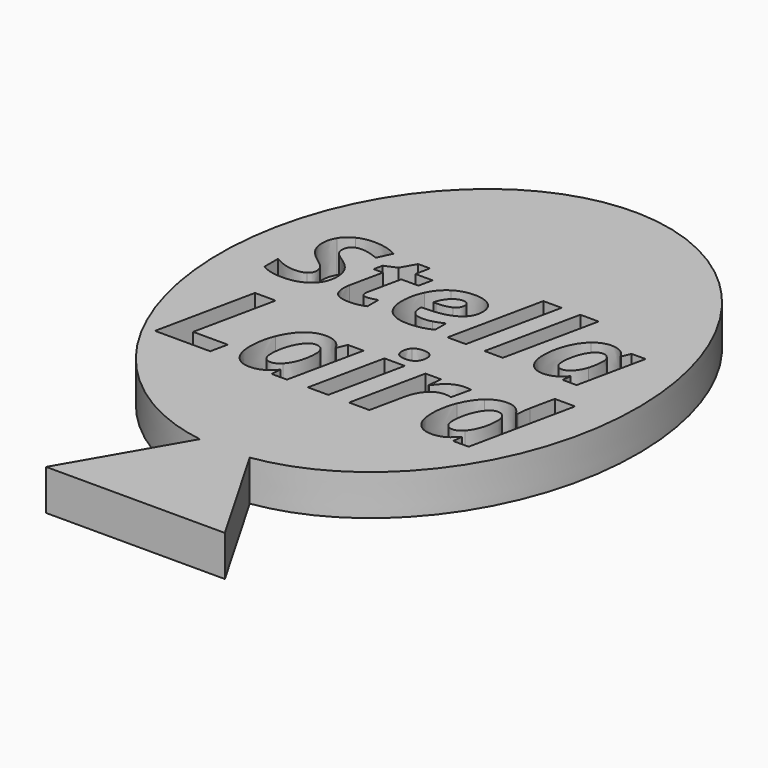
from build123d import *

# Parameters (mm, degrees)
F1_DEPTH       = 6.35
F0_TEXT_SIZE   = 19.5004373789
F0_TEXT_SIZE_2 = 21.6683653704
F2_DEPTH       = 1.27


# Not quite as in the source:
# - Text() gives the source's letters only with a copy of the font that has no kerning and outlines rounded to 1/6400 em; it was checked with that copy


with BuildPart() as f1:
    # F0 (on Top) → F1 (new body)
    with BuildSketch(Plane.XY):
        with BuildLine():
            add(Edge.make_bspline(
                [(3.9012639568, -39.93374284), (34.4777247718, -35.4132794138), (32.6371018831, 2.4039067683), (30.7964789943, 40.2210929505), (0, 40.2210929505)],
                knots=[3.2611985656, 3.2611985656, 3.2611985656, 4.7721919364, 4.7721919364, 6.2831853072, 6.2831853072, 6.2831853072], degree=2, weights=[1, 0.7279310805, 1, 0.7279310805, 1]))
            add(Edge.make_bspline(
                [(0, 40.2210929505), (-30.7964789943, 40.2210929505), (-32.6371018831, 2.4039067683), (-34.4777247718, -35.4132794138), (-3.9012639568, -39.93374284)],
                knots=[0, 0, 0, 1.5109933708, 1.5109933708, 3.0219867416, 3.0219867416, 3.0219867416], degree=2, weights=[1, 0.7279310805, 1, 0.7279310805, 1]))
            Line((-3.9012639568, -39.93374284), (0, -33.1765554531))
            Line((0, -33.1765554531), (3.9012639568, -39.93374284))
        make_face()
        Polygon((-17.4413733836, -20.9845771347), (-26.0850197571, -20.9845771347), (-22.8178365411, -5.5153956695), (-19.5777387818, -5.5153956695), (-22.2862844531, -18.2760314634), (-16.8691931105, -18.2760314634), align=None, mode=Mode.SUBTRACT)
        with BuildLine():
            add(Edge.make_bspline(
                [(-7.7481655624, -19.4508631483), (-9.1667663577, -21.1978751063), (-11.1236906053, -21.1978751063)],
                knots=[0, 0, 0, 1, 1, 1], degree=2))
            add(Edge.make_bspline(
                [(-11.1236906053, -21.1978751063), (-12.6811043662, -21.1978751063), (-13.5749244378, -20.0704429706)],
                knots=[0, 0, 0, 1, 1, 1], degree=2))
            add(Edge.make_bspline(
                [(-13.5749244378, -20.0704429706), (-14.4687445093, -18.943010835), (-14.4687445093, -16.9116015815)],
                knots=[0, 0, 0, 1, 1, 1], degree=2))
            add(Edge.make_bspline(
                [(-14.4687445093, -16.9116015815), (-14.4687445093, -14.8158643683), (-13.7069660393, -12.9164967163)],
                knots=[0, 0, 0, 1, 1, 1], degree=2))
            add(Edge.make_bspline(
                [(-13.7069660393, -12.9164967163), (-12.9451875692, -11.0171290643), (-11.7060279246, -9.9760318219)],
                knots=[0, 0, 0, 1, 1, 1], degree=2))
            add(Edge.make_bspline(
                [(-11.7060279246, -9.9760318219), (-10.46686828, -8.9349345795), (-8.987325207, -8.9349345795)],
                knots=[0, 0, 0, 1, 1, 1], degree=2))
            add(Edge.make_bspline(
                [(-8.987325207, -8.9349345795), (-7.961463534, -8.9349345795), (-7.2149206334, -9.3784589332)],
                knots=[0, 0, 0, 1, 1, 1], degree=2))
            add(Edge.make_bspline(
                [(-7.2149206334, -9.3784589332), (-6.4683777327, -9.8219832869), (-6.0553245178, -10.6684038092)],
                knots=[0, 0, 0, 1, 1, 1], degree=2))
            Line((-6.0553245178, -10.6684038092), (-5.9706824656, -10.6684038092))
            Line((-5.9706824656, -10.6684038092), (-5.3680310537, -9.1550039153))
            Line((-5.3680310537, -9.1550039153), (-2.9134115391, -9.1550039153))
            Line((-2.9134115391, -9.1550039153), (-5.4323590134, -20.9845771347))
            Line((-5.4323590134, -20.9845771347), (-7.8565073893, -20.9845771347))
            Line((-7.8565073893, -20.9845771347), (-7.7075373773, -19.4508631483))
            Line((-7.7075373773, -19.4508631483), (-7.7481655624, -19.4508631483))
        make_face(mode=Mode.SUBTRACT)
        Polygon((3.5396985227, -9.1550039153), (1.0309080947, -20.9845771347), (-2.1516330691, -20.9845771347), (0.3537716769, -9.1550039153), align=None, mode=Mode.SUBTRACT)
        with BuildLine():
            add(Edge.make_bspline(
                [(9.0617460101, -11.345540227), (10.6191597711, -8.9349345795), (12.7961533544, -8.9349345795)],
                knots=[0, 0, 0, 1, 1, 1], degree=2))
            add(Edge.make_bspline(
                [(12.7961533544, -8.9349345795), (13.4225045409, -8.9349345795), (13.8118579811, -9.0500477706)],
                knots=[0, 0, 0, 1, 1, 1], degree=2))
            Line((13.8118579811, -9.0500477706), (13.1144074708, -12.1174757433))
            add(Edge.make_bspline(
                [(13.1144074708, -12.1174757433), (12.6370262962, -11.9481916388), (12.058074659, -11.9481916388)],
                knots=[0, 0, 0, 1, 1, 1], degree=2))
            add(Edge.make_bspline(
                [(12.058074659, -11.9481916388), (10.8290720606, -11.9481916388), (9.9030880092, -12.9164967163)],
                knots=[0, 0, 0, 1, 1, 1], degree=2))
            add(Edge.make_bspline(
                [(9.9030880092, -12.9164967163), (8.9771039579, -13.8848017938), (8.5877505176, -15.6927560294)],
                knots=[0, 0, 0, 1, 1, 1], degree=2))
            Line((8.5877505176, -15.6927560294), (7.463704064, -20.9845771347))
            Line((7.463704064, -20.9845771347), (4.2811629002, -20.9845771347))
            Line((4.2811629002, -20.9845771347), (6.7865676462, -9.1550039153))
            Line((6.7865676462, -9.1550039153), (9.2208730683, -9.1550039153))
            Line((9.2208730683, -9.1550039153), (8.9974180504, -11.345540227))
            Line((8.9974180504, -11.345540227), (9.0617460101, -11.345540227))
        make_face(mode=Mode.SUBTRACT)
        with BuildLine():
            add(Edge.make_bspline(
                [(19.1087576095, -20.7848218915), (18.2877297029, -21.1978751063), (17.3058818971, -21.1978751063)],
                knots=[0, 0, 0, 1, 1, 1], degree=2))
            add(Edge.make_bspline(
                [(17.3058818971, -21.1978751063), (15.7484681361, -21.1978751063), (14.8546480646, -20.0653644475)],
                knots=[0, 0, 0, 1, 1, 1], degree=2))
            add(Edge.make_bspline(
                [(14.8546480646, -20.0653644475), (13.960827993, -18.9328537887), (13.960827993, -16.891287489)],
                knots=[0, 0, 0, 1, 1, 1], degree=2))
            add(Edge.make_bspline(
                [(13.960827993, -16.891287489), (13.960827993, -14.8158643683), (14.71752794, -12.9266537626)],
                knots=[0, 0, 0, 1, 1, 1], degree=2))
            add(Edge.make_bspline(
                [(14.71752794, -12.9266537626), (15.4742278869, -11.0374431569), (16.7116946904, -9.9861888682)],
                knots=[0, 0, 0, 1, 1, 1], degree=2))
            add(Edge.make_bspline(
                [(16.7116946904, -9.9861888682), (17.949161494, -8.9349345795), (19.4422472953, -8.9349345795)],
                knots=[0, 0, 0, 1, 1, 1], degree=2))
            add(Edge.make_bspline(
                [(19.4422472953, -8.9349345795), (20.3089819101, -8.9349345795), (20.9387187787, -9.3259808608)],
                knots=[0, 0, 0, 1, 1, 1], degree=2))
            add(Edge.make_bspline(
                [(20.9387187787, -9.3259808608), (21.5684556473, -9.7170271421), (22.1304788741, -10.6684038092)],
                knots=[0, 0, 0, 1, 1, 1], degree=2))
            Line((22.1304788741, -10.6684038092), (22.2151209263, -10.6684038092))
            Line((22.2151209263, -10.6684038092), (22.2354350188, -10.3738494674))
            add(Edge.make_bspline(
                [(22.2354350188, -10.3738494674), (22.2997629785, -9.2091748288), (22.4995182218, -8.308583393)],
                knots=[0, 0, 0, 1, 1, 1], degree=2))
            Line((22.4995182218, -8.308583393), (23.305310559, -4.5200051353))
            Line((23.305310559, -4.5200051353), (26.4878517228, -4.5200051353))
            Line((26.4878517228, -4.5200051353), (22.9972134889, -20.9845771347))
            Line((22.9972134889, -20.9845771347), (20.5730651131, -20.9845771347))
            Line((20.5730651131, -20.9845771347), (20.722035125, -19.4508631483))
            Line((20.722035125, -19.4508631483), (20.6814069399, -19.4508631483))
            add(Edge.make_bspline(
                [(20.6814069399, -19.4508631483), (19.9297855162, -20.3717686766), (19.1087576095, -20.7848218915)],
                knots=[0, 0, 0, 1, 1, 1], degree=2))
        make_face(mode=Mode.SUBTRACT)
        with BuildLine():
            add(Edge.make_bspline(
                [(-18.2115803458, 6.2599450929), (-17.6402784695, 5.3412916758), (-17.6402784695, 4.1133735096)],
                knots=[0, 0, 0, 1, 1, 1], degree=2))
            add(Edge.make_bspline(
                [(-17.6402784695, 4.1133735096), (-17.6402784695, 2.1237195083), (-19.0494897645, 0.9658810389)],
                knots=[0, 0, 0, 1, 1, 1], degree=2))
            add(Edge.make_bspline(
                [(-19.0494897645, 0.9658810389), (-20.4587010594, -0.1919574304), (-22.8657862984, -0.1919574304)],
                knots=[0, 0, 0, 1, 1, 1], degree=2))
            add(Edge.make_bspline(
                [(-22.8657862984, -0.1919574304), (-24.9712241466, -0.1919574304), (-26.2570342363, 0.6672805916)],
                knots=[0, 0, 0, 1, 1, 1], degree=2))
            Line((-26.2570342363, 0.6672805916), (-26.2570342363, 3.275464091))
            add(Edge.make_bspline(
                [(-26.2570342363, 3.275464091), (-24.419727402, 2.2486441852), (-22.8475046383, 2.2486441852)],
                knots=[0, 0, 0, 1, 1, 1], degree=2))
            add(Edge.make_bspline(
                [(-22.8475046383, 2.2486441852), (-21.7810744692, 2.2486441852), (-21.1808266311, 2.6523641779)],
                knots=[0, 0, 0, 1, 1, 1], degree=2))
            add(Edge.make_bspline(
                [(-21.1808266311, 2.6523641779), (-20.580578793, 3.0560841705), (-20.580578793, 3.7599280821)],
                knots=[0, 0, 0, 1, 1, 1], degree=2))
            add(Edge.make_bspline(
                [(-20.580578793, 3.7599280821), (-20.580578793, 4.1712654331), (-20.710073885, 4.4805301821)],
                knots=[0, 0, 0, 1, 1, 1], degree=2))
            add(Edge.make_bspline(
                [(-20.710073885, 4.4805301821), (-20.839568977, 4.7897949312), (-21.0772305575, 5.0564024735)],
                knots=[0, 0, 0, 1, 1, 1], degree=2))
            add(Edge.make_bspline(
                [(-21.0772305575, 5.0564024735), (-21.3148921381, 5.3230100158), (-22.2563976303, 6.0268539274)],
                knots=[0, 0, 0, 1, 1, 1], degree=2))
            add(Edge.make_bspline(
                [(-22.2563976303, 6.0268539274), (-23.5726771534, 6.9714063629), (-24.1058922379, 7.8946301951)],
                knots=[0, 0, 0, 1, 1, 1], degree=2))
            add(Edge.make_bspline(
                [(-24.1058922379, 7.8946301951), (-24.6391073225, 8.8178540273), (-24.6391073225, 9.8842841964)],
                knots=[0, 0, 0, 1, 1, 1], degree=2))
            add(Edge.make_bspline(
                [(-24.6391073225, 9.8842841964), (-24.6391073225, 11.1122023626), (-24.0480003145, 12.0780834015)],
                knots=[0, 0, 0, 1, 1, 1], degree=2))
            add(Edge.make_bspline(
                [(-24.0480003145, 12.0780834015), (-23.4568933064, 13.0439644404), (-22.3660875905, 13.58174994)],
                knots=[0, 0, 0, 1, 1, 1], degree=2))
            add(Edge.make_bspline(
                [(-22.3660875905, 13.58174994), (-21.2752818747, 14.1195354396), (-19.8584532214, 14.1195354396)],
                knots=[0, 0, 0, 1, 1, 1], degree=2))
            add(Edge.make_bspline(
                [(-19.8584532214, 14.1195354396), (-17.7926256365, 14.1195354396), (-16.0771965359, 13.1780299474)],
                knots=[0, 0, 0, 1, 1, 1], degree=2))
            Line((-16.0771965359, 13.1780299474), (-17.116204215, 10.9598551956))
            add(Edge.make_bspline(
                [(-17.116204215, 10.9598551956), (-18.6000656218, 11.6636991072), (-19.8584532214, 11.6636991072)],
                knots=[0, 0, 0, 1, 1, 1], degree=2))
            add(Edge.make_bspline(
                [(-19.8584532214, 11.6636991072), (-20.6476115465, 11.6636991072), (-21.1518806694, 11.2356035679)],
                knots=[0, 0, 0, 1, 1, 1], degree=2))
            add(Edge.make_bspline(
                [(-21.1518806694, 11.2356035679), (-21.6561497922, 10.8075080286), (-21.6561497922, 10.1036641169)],
                knots=[0, 0, 0, 1, 1, 1], degree=2))
            add(Edge.make_bspline(
                [(-21.6561497922, 10.1036641169), (-21.6561497922, 9.5216979389), (-21.3423146282, 9.0890319846)],
                knots=[0, 0, 0, 1, 1, 1], degree=2))
            add(Edge.make_bspline(
                [(-21.3423146282, 9.0890319846), (-21.0284794641, 8.6563660302), (-19.9346268049, 7.9403343452)],
                knots=[0, 0, 0, 1, 1, 1], degree=2))
            add(Edge.make_bspline(
                [(-19.9346268049, 7.9403343452), (-18.7828822222, 7.1785985101), (-18.2115803458, 6.2599450929)],
                knots=[0, 0, 0, 1, 1, 1], degree=2))
        make_face(mode=Mode.SUBTRACT)
        with BuildLine():
            add(Edge.make_bspline(
                [(-12.2593765303, 2.8275634199), (-12.2593765303, 2.1237195083), (-11.4214671117, 2.1237195083)],
                knots=[0, 0, 0, 1, 1, 1], degree=2))
            add(Edge.make_bspline(
                [(-11.4214671117, 2.1237195083), (-10.8029376136, 2.1237195083), (-9.8766668381, 2.4558363324)],
                knots=[0, 0, 0, 1, 1, 1], degree=2))
            Line((-9.8766668381, 2.4558363324), (-9.8766668381, 0.3138351641))
            add(Edge.make_bspline(
                [(-9.8766668381, 0.3138351641), (-10.9339561772, -0.1919574304), (-12.4117236973, -0.1919574304)],
                knots=[0, 0, 0, 1, 1, 1], degree=2))
            add(Edge.make_bspline(
                [(-12.4117236973, -0.1919574304), (-13.8376931806, -0.1919574304), (-14.5095441872, 0.4082904076)],
                knots=[0, 0, 0, 1, 1, 1], degree=2))
            add(Edge.make_bspline(
                [(-14.5095441872, 0.4082904076), (-15.1813951938, 1.0085382457), (-15.1813951938, 2.2669258453)],
                knots=[0, 0, 0, 1, 1, 1], degree=2))
            add(Edge.make_bspline(
                [(-15.1813951938, 2.2669258453), (-15.1813951938, 2.7422490064), (-15.0686582902, 3.3333560144)],
                knots=[0, 0, 0, 1, 1, 1], degree=2))
            Line((-15.0686582902, 3.3333560144), (-13.9717586876, 8.4644085998))
            Line((-13.9717586876, 8.4644085998), (-15.4190567743, 8.4644085998))
            Line((-15.4190567743, 8.4644085998), (-15.1448318737, 9.8660025364))
            Line((-15.1448318737, 9.8660025364), (-13.277055606, 10.6643016916))
            Line((-13.277055606, 10.6643016916), (-12.0217149497, 12.9129458768))
            Line((-12.0217149497, 12.9129458768), (-10.1722203421, 12.9129458768))
            Line((-10.1722203421, 12.9129458768), (-10.6384026732, 10.6460200315))
            Line((-10.6384026732, 10.6460200315), (-7.9449047602, 10.6460200315))
            Line((-7.9449047602, 10.6460200315), (-8.4202279213, 8.4644085998))
            Line((-8.4202279213, 8.4644085998), (-11.1076319476, 8.4644085998))
            Line((-11.1076319476, 8.4644085998), (-12.2014846068, 3.3333560144))
            add(Edge.make_bspline(
                [(-12.2014846068, 3.3333560144), (-12.2593765303, 3.0469433404), (-12.2593765303, 2.8275634199)],
                knots=[0, 0, 0, 1, 1, 1], degree=2))
        make_face(mode=Mode.SUBTRACT)
        with BuildLine():
            add(Edge.make_bspline(
                [(0.4616119161, 0.6276703281), (-1.1745966577, -0.1919574304), (-3.2495650726, -0.1919574304)],
                knots=[0, 0, 0, 1, 1, 1], degree=2))
            add(Edge.make_bspline(
                [(-3.2495650726, -0.1919574304), (-5.2514068473, -0.1919574304), (-6.3559238082, 0.8851370404)],
                knots=[0, 0, 0, 1, 1, 1], degree=2))
            add(Edge.make_bspline(
                [(-6.3559238082, 0.8851370404), (-7.4604407691, 1.9622315112), (-7.4604407691, 3.9244630225)],
                knots=[0, 0, 0, 1, 1, 1], degree=2))
            add(Edge.make_bspline(
                [(-7.4604407691, 3.9244630225), (-7.4604407691, 5.8927884204), (-6.6743293872, 7.5168092209)],
                knots=[0, 0, 0, 1, 1, 1], degree=2))
            add(Edge.make_bspline(
                [(-6.6743293872, 7.5168092209), (-5.8882180054, 9.1408300213), (-4.5460394639, 9.992450685)],
                knots=[0, 0, 0, 1, 1, 1], degree=2))
            add(Edge.make_bspline(
                [(-4.5460394639, 9.992450685), (-3.2038609225, 10.8440713486), (-1.5097604252, 10.8440713486)],
                knots=[0, 0, 0, 1, 1, 1], degree=2))
            add(Edge.make_bspline(
                [(-1.5097604252, 10.8440713486), (0.1782461854, 10.8440713486), (1.1197516776, 10.0686242685)],
                knots=[0, 0, 0, 1, 1, 1], degree=2))
            add(Edge.make_bspline(
                [(1.1197516776, 10.0686242685), (2.0612571698, 9.2931771884), (2.0612571698, 7.9403343452)],
                knots=[0, 0, 0, 1, 1, 1], degree=2))
            add(Edge.make_bspline(
                [(2.0612571698, 7.9403343452), (2.0612571698, 6.1609194344), (0.4722762178, 5.1950383955)],
                knots=[0, 0, 0, 1, 1, 1], degree=2))
            add(Edge.make_bspline(
                [(0.4722762178, 5.1950383955), (-1.1167047343, 4.2291573565), (-4.0691928312, 4.2291573565)],
                knots=[0, 0, 0, 1, 1, 1], degree=2))
            Line((-4.0691928312, 4.2291573565), (-4.5567037656, 4.2291573565))
            Line((-4.5567037656, 4.2291573565), (-4.5749854257, 4.0280590961))
            Line((-4.5749854257, 4.0280590961), (-4.5749854257, 3.8361016656))
            add(Edge.make_bspline(
                [(-4.5749854257, 3.8361016656), (-4.5749854257, 2.9707697569), (-4.0844275479, 2.4710710491)],
                knots=[0, 0, 0, 1, 1, 1], degree=2))
            add(Edge.make_bspline(
                [(-4.0844275479, 2.4710710491), (-3.5938696701, 1.9713723413), (-2.6797866679, 1.9713723413)],
                knots=[0, 0, 0, 1, 1, 1], degree=2))
            add(Edge.make_bspline(
                [(-2.6797866679, 1.9713723413), (-1.8510180793, 1.9713723413), (-1.1745966577, 2.15266547)],
                knots=[0, 0, 0, 1, 1, 1], degree=2))
            add(Edge.make_bspline(
                [(-1.1745966577, 2.15266547), (-0.4981752362, 2.3339585988), (0.4616119161, 2.7910000998)],
                knots=[0, 0, 0, 1, 1, 1], degree=2))
            Line((0.4616119161, 2.7910000998), (0.4616119161, 0.6276703281))
        make_face(mode=Mode.SUBTRACT)
        with BuildLine():
            add(Edge.make_bspline(
                [(2.4596659363, -7.6856178886), (0.8616239902, -7.6856178886), (0.8616239902, -6.3821302843)],
                knots=[0, 0, 0, 1, 1, 1], degree=2))
            add(Edge.make_bspline(
                [(0.8616239902, -6.3821302843), (0.8616239902, -5.4646104382), (1.3643977805, -4.9923077868)],
                knots=[0, 0, 0, 1, 1, 1], degree=2))
            add(Edge.make_bspline(
                [(1.3643977805, -4.9923077868), (1.8671715707, -4.5200051353), (2.7880770989, -4.5200051353)],
                knots=[0, 0, 0, 1, 1, 1], degree=2))
            add(Edge.make_bspline(
                [(2.7880770989, -4.5200051353), (3.5600126153, -4.5200051353), (3.9629087839, -4.848416298)],
                knots=[0, 0, 0, 1, 1, 1], degree=2))
            add(Edge.make_bspline(
                [(3.9629087839, -4.848416298), (4.3658049525, -5.1768274606), (4.3658049525, -5.7896359187)],
                knots=[0, 0, 0, 1, 1, 1], degree=2))
            add(Edge.make_bspline(
                [(4.3658049525, -5.7896359187), (4.3658049525, -6.636056441), (3.9002736652, -7.1608371648)],
                knots=[0, 0, 0, 1, 1, 1], degree=2))
            add(Edge.make_bspline(
                [(3.9002736652, -7.1608371648), (3.434742378, -7.6856178886), (2.4596659363, -7.6856178886)],
                knots=[0, 0, 0, 1, 1, 1], degree=2))
        make_face(mode=Mode.SUBTRACT)
        Polygon((8.9107857991, 14.8172854646), (5.7663402718, 0), (2.9022135318, 0), (6.0436121158, 14.8172854646), align=None, mode=Mode.SUBTRACT)
        Polygon((14.699978146, 14.8172854646), (11.5555326186, 0), (8.6914058786, 0), (11.8328044626, 14.8172854646), align=None, mode=Mode.SUBTRACT)
        with BuildLine():
            add(Edge.make_bspline(
                [(21.0315264074, 1.3802653332), (19.7548571478, -0.1919574304), (17.993723897, -0.1919574304)],
                knots=[0, 0, 0, 1, 1, 1], degree=2))
            add(Edge.make_bspline(
                [(17.993723897, -0.1919574304), (16.5921299604, -0.1919574304), (15.7877369185, 0.8226747019)],
                knots=[0, 0, 0, 1, 1, 1], degree=2))
            add(Edge.make_bspline(
                [(15.7877369185, 0.8226747019), (14.9833438766, 1.8373068343), (14.9833438766, 3.6654728386)],
                knots=[0, 0, 0, 1, 1, 1], degree=2))
            add(Edge.make_bspline(
                [(14.9833438766, 3.6654728386), (14.9833438766, 5.5515307663), (15.6689061282, 7.2608659803)],
                knots=[0, 0, 0, 1, 1, 1], degree=2))
            add(Edge.make_bspline(
                [(15.6689061282, 7.2608659803), (16.3544683798, 8.9702011943), (17.4696496424, 9.9071362715)],
                knots=[0, 0, 0, 1, 1, 1], degree=2))
            add(Edge.make_bspline(
                [(17.4696496424, 9.9071362715), (18.5848309051, 10.8440713486), (19.9163451448, 10.8440713486)],
                knots=[0, 0, 0, 1, 1, 1], degree=2))
            add(Edge.make_bspline(
                [(19.9163451448, 10.8440713486), (20.839568977, 10.8440713486), (21.5114199835, 10.444921771)],
                knots=[0, 0, 0, 1, 1, 1], degree=2))
            add(Edge.make_bspline(
                [(21.5114199835, 10.444921771), (22.1832709901, 10.0457721935), (22.5549980777, 9.2840363583)],
                knots=[0, 0, 0, 1, 1, 1], degree=2))
            Line((22.5549980777, 9.2840363583), (22.6311716612, 9.2840363583))
            Line((22.6311716612, 9.2840363583), (23.1735275758, 10.6460200315))
            Line((23.1735275758, 10.6460200315), (25.3825614976, 10.6460200315))
            Line((25.3825614976, 10.6460200315), (23.1156356523, 0))
            Line((23.1156356523, 0), (20.9340242205, 0))
            Line((20.9340242205, 0), (21.0680897275, 1.3802653332))
            Line((21.0680897275, 1.3802653332), (21.0315264074, 1.3802653332))
        make_face(mode=Mode.SUBTRACT)
        with BuildLine():
            add(Edge.make_bspline(
                [(-3.9012639568, -39.93374284), (0, -40.510510738), (3.9012639568, -39.93374284)],
                knots=[3.0219867416, 3.0219867416, 3.0219867416, 3.2611985656, 3.2611985656, 3.2611985656], degree=2, weights=[1, 0.9928557359, 1]))
            Line((-3.9012639568, -39.93374284), (-13.9888415253, -57.4059397139))
            Line((-13.9888415253, -57.4059397139), (13.9888415253, -57.4059397139))
            Line((13.9888415253, -57.4059397139), (3.9012639568, -39.93374284))
        make_face()
        with BuildLine():
            Line((0, -33.1765554531), (-3.9012639568, -39.93374284))
            add(Edge.make_bspline(
                [(-3.9012639568, -39.93374284), (0, -40.510510738), (3.9012639568, -39.93374284)],
                knots=[3.0219867416, 3.0219867416, 3.0219867416, 3.2611985656, 3.2611985656, 3.2611985656], degree=2, weights=[1, 0.9928557359, 1]))
            Line((3.9012639568, -39.93374284), (0, -33.1765554531))
        make_face()
    extrude(amount=F1_DEPTH)



with BuildPart() as f1b:
    # F0 (on Top) → F1, piece 2 (new body)
    with BuildSketch(Plane.XY):
        with BuildLine():
            add(Edge.make_bspline(
                [(-0.6901326666, 7.8733015917), (-0.6901326666, 8.7782437638), (-1.6895300823, 8.7782437638)],
                knots=[0, 0, 0, 1, 1, 1], degree=2))
            add(Edge.make_bspline(
                [(-1.6895300823, 8.7782437638), (-2.5274395009, 8.7782437638), (-3.2693702043, 8.0165079287)],
                knots=[0, 0, 0, 1, 1, 1], degree=2))
            add(Edge.make_bspline(
                [(-3.2693702043, 8.0165079287), (-4.0113009077, 7.2547720936), (-4.2398216582, 6.1609194344)],
                knots=[0, 0, 0, 1, 1, 1], degree=2))
            Line((-4.2398216582, 6.1609194344), (-3.8132495906, 6.1609194344))
            add(Edge.make_bspline(
                [(-3.8132495906, 6.1609194344), (-2.3354820705, 6.1609194344), (-1.5128073685, 6.6225313505)],
                knots=[0, 0, 0, 1, 1, 1], degree=2))
            add(Edge.make_bspline(
                [(-1.5128073685, 6.6225313505), (-0.6901326666, 7.0841432665), (-0.6901326666, 7.8733015917)],
                knots=[0, 0, 0, 1, 1, 1], degree=2))
        make_face()
    extrude(amount=F1_DEPTH)


with BuildPart() as f1c:
    # F0 (on Top) → F1, piece 3 (new body)
    with BuildSketch(Plane.XY):
        with BuildLine():
            add(Edge.make_bspline(
                [(18.2070099308, 2.5426742176), (18.5269389816, 2.1237195083), (19.1180459896, 2.1237195083)],
                knots=[0, 0, 0, 1, 1, 1], degree=2))
            add(Edge.make_bspline(
                [(19.1180459896, 2.1237195083), (19.7731388078, 2.1237195083), (20.3825274759, 2.7620541381)],
                knots=[0, 0, 0, 1, 1, 1], degree=2))
            add(Edge.make_bspline(
                [(20.3825274759, 2.7620541381), (20.991916144, 3.4003887679), (21.3636432315, 4.4896710121)],
                knots=[0, 0, 0, 1, 1, 1], degree=2))
            add(Edge.make_bspline(
                [(21.3636432315, 4.4896710121), (21.7353703191, 5.5789532564), (21.7353703191, 6.9592185896)],
                knots=[0, 0, 0, 1, 1, 1], degree=2))
            add(Edge.make_bspline(
                [(21.7353703191, 6.9592185896), (21.7353703191, 7.6356400112), (21.3682136465, 8.0789702672)],
                knots=[0, 0, 0, 1, 1, 1], degree=2))
            add(Edge.make_bspline(
                [(21.3682136465, 8.0789702672), (21.001056974, 8.5223005232), (20.400809136, 8.5223005232)],
                knots=[0, 0, 0, 1, 1, 1], degree=2))
            add(Edge.make_bspline(
                [(20.400809136, 8.5223005232), (19.7548571478, 8.5223005232), (19.1698440264, 7.8367382716)],
                knots=[0, 0, 0, 1, 1, 1], degree=2))
            add(Edge.make_bspline(
                [(19.1698440264, 7.8367382716), (18.5848309051, 7.15117602), (18.2359558926, 6.0268539274)],
                knots=[0, 0, 0, 1, 1, 1], degree=2))
            add(Edge.make_bspline(
                [(18.2359558926, 6.0268539274), (17.8870808801, 4.9025318348), (17.8870808801, 3.7995383455)],
                knots=[0, 0, 0, 1, 1, 1], degree=2))
            add(Edge.make_bspline(
                [(17.8870808801, 3.7995383455), (17.8870808801, 2.9616289269), (18.2070099308, 2.5426742176)],
                knots=[0, 0, 0, 1, 1, 1], degree=2))
        make_face()
    extrude(amount=F1_DEPTH)


with BuildPart() as f1d:
    # F0 (on Top) → F1, piece 4 (new body)
    with BuildSketch(Plane.XY):
        with BuildLine():
            add(Edge.make_bspline(
                [(-10.886692859, -18.1592254313), (-10.5311962397, -18.6247567186), (-9.8743739144, -18.6247567186)],
                knots=[0, 0, 0, 1, 1, 1], degree=2))
            add(Edge.make_bspline(
                [(-9.8743739144, -18.6247567186), (-9.1464522652, -18.6247567186), (-8.4693158474, -17.9154563209)],
                knots=[0, 0, 0, 1, 1, 1], degree=2))
            add(Edge.make_bspline(
                [(-8.4693158474, -17.9154563209), (-7.7921794296, -17.2061559233), (-7.3791262147, -15.9957745764)],
                knots=[0, 0, 0, 1, 1, 1], degree=2))
            add(Edge.make_bspline(
                [(-7.3791262147, -15.9957745764), (-6.9660729998, -14.7853932295), (-6.9660729998, -13.2516792432)],
                knots=[0, 0, 0, 1, 1, 1], degree=2))
            add(Edge.make_bspline(
                [(-6.9660729998, -13.2516792432), (-6.9660729998, -12.5000578194), (-7.3740476916, -12.0074410754)],
                knots=[0, 0, 0, 1, 1, 1], degree=2))
            add(Edge.make_bspline(
                [(-7.3740476916, -12.0074410754), (-7.7820223833, -11.5148243314), (-8.4490017548, -11.5148243314)],
                knots=[0, 0, 0, 1, 1, 1], degree=2))
            add(Edge.make_bspline(
                [(-8.4490017548, -11.5148243314), (-9.1667663577, -11.5148243314), (-9.8168173189, -12.2766028015)],
                knots=[0, 0, 0, 1, 1, 1], degree=2))
            add(Edge.make_bspline(
                [(-9.8168173189, -12.2766028015), (-10.46686828, -13.0383812715), (-10.8545288792, -14.2876979624)],
                knots=[0, 0, 0, 1, 1, 1], degree=2))
            add(Edge.make_bspline(
                [(-10.8545288792, -14.2876979624), (-11.2421894784, -15.5370146533), (-11.2421894784, -16.7626315696)],
                knots=[0, 0, 0, 1, 1, 1], degree=2))
            add(Edge.make_bspline(
                [(-11.2421894784, -16.7626315696), (-11.2421894784, -17.6936941441), (-10.886692859, -18.1592254313)],
                knots=[0, 0, 0, 1, 1, 1], degree=2))
        make_face()
    extrude(amount=F1_DEPTH)


with BuildPart() as f1e:
    # F0 (on Top) → F1, piece 5 (new body)
    with BuildSketch(Plane.XY):
        with BuildLine():
            add(Edge.make_bspline(
                [(17.187383024, -16.7626315696), (17.187383024, -18.6247567186), (18.6398406402, -18.6247567186)],
                knots=[0, 0, 0, 1, 1, 1], degree=2))
            add(Edge.make_bspline(
                [(18.6398406402, -18.6247567186), (19.3372911506, -18.6247567186), (19.9974991579, -17.9002207515)],
                knots=[0, 0, 0, 1, 1, 1], degree=2))
            add(Edge.make_bspline(
                [(19.9974991579, -17.9002207515), (20.6577071653, -17.1756847845), (21.0606033339, -15.9686891197)],
                knots=[0, 0, 0, 1, 1, 1], degree=2))
            add(Edge.make_bspline(
                [(21.0606033339, -15.9686891197), (21.4634995025, -14.7616934549), (21.4634995025, -13.3769494805)],
                knots=[0, 0, 0, 1, 1, 1], degree=2))
            add(Edge.make_bspline(
                [(21.4634995025, -13.3769494805), (21.4634995025, -12.5305289582), (21.0673746981, -12.0226766448)],
                knots=[0, 0, 0, 1, 1, 1], degree=2))
            add(Edge.make_bspline(
                [(21.0673746981, -12.0226766448), (20.6712498937, -11.5148243314), (19.9805707475, -11.5148243314)],
                knots=[0, 0, 0, 1, 1, 1], degree=2))
            add(Edge.make_bspline(
                [(19.9805707475, -11.5148243314), (19.2628061446, -11.5148243314), (18.6127551835, -12.2766028015)],
                knots=[0, 0, 0, 1, 1, 1], degree=2))
            add(Edge.make_bspline(
                [(18.6127551835, -12.2766028015), (17.9627042224, -13.0383812715), (17.5750436232, -14.2876979624)],
                knots=[0, 0, 0, 1, 1, 1], degree=2))
            add(Edge.make_bspline(
                [(17.5750436232, -14.2876979624), (17.187383024, -15.5370146533), (17.187383024, -16.7626315696)],
                knots=[0, 0, 0, 1, 1, 1], degree=2))
        make_face()
    extrude(amount=F1_DEPTH)


with BuildPart() as f1_1:
    add(f1.part)

    add(f1b.part)  # F2 merges F1b

    add(f1c.part)  # F2 merges F1c

    add(f1d.part)  # F2 merges F1d

    add(f1e.part)  # F2 merges F1e
    # F0 (on Top) → F2 (join)
    with BuildSketch(Plane.XY):
        with Locations((-26.6470429839, 0)):
            Text('Stella', F0_TEXT_SIZE, font='Open Sans', font_style=FontStyle.BOLDITALIC, text_align=(TextAlign.LEFT, TextAlign.BOTTOM))
        with BuildLine():
            add(Edge.make_bspline(
                [(-10.886692859, -18.1592254313), (-10.5311962397, -18.6247567186), (-9.8743739144, -18.6247567186)],
                knots=[0, 0, 0, 1, 1, 1], degree=2))
            add(Edge.make_bspline(
                [(-9.8743739144, -18.6247567186), (-9.1464522652, -18.6247567186), (-8.4693158474, -17.9154563209)],
                knots=[0, 0, 0, 1, 1, 1], degree=2))
            add(Edge.make_bspline(
                [(-8.4693158474, -17.9154563209), (-7.7921794296, -17.2061559233), (-7.3791262147, -15.9957745764)],
                knots=[0, 0, 0, 1, 1, 1], degree=2))
            add(Edge.make_bspline(
                [(-7.3791262147, -15.9957745764), (-6.9660729998, -14.7853932295), (-6.9660729998, -13.2516792432)],
                knots=[0, 0, 0, 1, 1, 1], degree=2))
            add(Edge.make_bspline(
                [(-6.9660729998, -13.2516792432), (-6.9660729998, -12.5000578194), (-7.3740476916, -12.0074410754)],
                knots=[0, 0, 0, 1, 1, 1], degree=2))
            add(Edge.make_bspline(
                [(-7.3740476916, -12.0074410754), (-7.7820223833, -11.5148243314), (-8.4490017548, -11.5148243314)],
                knots=[0, 0, 0, 1, 1, 1], degree=2))
            add(Edge.make_bspline(
                [(-8.4490017548, -11.5148243314), (-9.1667663577, -11.5148243314), (-9.8168173189, -12.2766028015)],
                knots=[0, 0, 0, 1, 1, 1], degree=2))
            add(Edge.make_bspline(
                [(-9.8168173189, -12.2766028015), (-10.46686828, -13.0383812715), (-10.8545288792, -14.2876979624)],
                knots=[0, 0, 0, 1, 1, 1], degree=2))
            add(Edge.make_bspline(
                [(-10.8545288792, -14.2876979624), (-11.2421894784, -15.5370146533), (-11.2421894784, -16.7626315696)],
                knots=[0, 0, 0, 1, 1, 1], degree=2))
            add(Edge.make_bspline(
                [(-11.2421894784, -16.7626315696), (-11.2421894784, -17.6936941441), (-10.886692859, -18.1592254313)],
                knots=[0, 0, 0, 1, 1, 1], degree=2))
        make_face()
        with Locations((-26.6470429839, -20.9845771347)):
            Text('Laird', F0_TEXT_SIZE_2, font='Open Sans', font_style=FontStyle.BOLDITALIC, text_align=(TextAlign.LEFT, TextAlign.BOTTOM))
        with BuildLine():
            add(Edge.make_bspline(
                [(17.187383024, -16.7626315696), (17.187383024, -18.6247567186), (18.6398406402, -18.6247567186)],
                knots=[0, 0, 0, 1, 1, 1], degree=2))
            add(Edge.make_bspline(
                [(18.6398406402, -18.6247567186), (19.3372911506, -18.6247567186), (19.9974991579, -17.9002207515)],
                knots=[0, 0, 0, 1, 1, 1], degree=2))
            add(Edge.make_bspline(
                [(19.9974991579, -17.9002207515), (20.6577071653, -17.1756847845), (21.0606033339, -15.9686891197)],
                knots=[0, 0, 0, 1, 1, 1], degree=2))
            add(Edge.make_bspline(
                [(21.0606033339, -15.9686891197), (21.4634995025, -14.7616934549), (21.4634995025, -13.3769494805)],
                knots=[0, 0, 0, 1, 1, 1], degree=2))
            add(Edge.make_bspline(
                [(21.4634995025, -13.3769494805), (21.4634995025, -12.5305289582), (21.0673746981, -12.0226766448)],
                knots=[0, 0, 0, 1, 1, 1], degree=2))
            add(Edge.make_bspline(
                [(21.0673746981, -12.0226766448), (20.6712498937, -11.5148243314), (19.9805707475, -11.5148243314)],
                knots=[0, 0, 0, 1, 1, 1], degree=2))
            add(Edge.make_bspline(
                [(19.9805707475, -11.5148243314), (19.2628061446, -11.5148243314), (18.6127551835, -12.2766028015)],
                knots=[0, 0, 0, 1, 1, 1], degree=2))
            add(Edge.make_bspline(
                [(18.6127551835, -12.2766028015), (17.9627042224, -13.0383812715), (17.5750436232, -14.2876979624)],
                knots=[0, 0, 0, 1, 1, 1], degree=2))
            add(Edge.make_bspline(
                [(17.5750436232, -14.2876979624), (17.187383024, -15.5370146533), (17.187383024, -16.7626315696)],
                knots=[0, 0, 0, 1, 1, 1], degree=2))
        make_face()
        with BuildLine():
            add(Edge.make_bspline(
                [(18.2070099308, 2.5426742176), (18.5269389816, 2.1237195083), (19.1180459896, 2.1237195083)],
                knots=[0, 0, 0, 1, 1, 1], degree=2))
            add(Edge.make_bspline(
                [(19.1180459896, 2.1237195083), (19.7731388078, 2.1237195083), (20.3825274759, 2.7620541381)],
                knots=[0, 0, 0, 1, 1, 1], degree=2))
            add(Edge.make_bspline(
                [(20.3825274759, 2.7620541381), (20.991916144, 3.4003887679), (21.3636432315, 4.4896710121)],
                knots=[0, 0, 0, 1, 1, 1], degree=2))
            add(Edge.make_bspline(
                [(21.3636432315, 4.4896710121), (21.7353703191, 5.5789532564), (21.7353703191, 6.9592185896)],
                knots=[0, 0, 0, 1, 1, 1], degree=2))
            add(Edge.make_bspline(
                [(21.7353703191, 6.9592185896), (21.7353703191, 7.6356400112), (21.3682136465, 8.0789702672)],
                knots=[0, 0, 0, 1, 1, 1], degree=2))
            add(Edge.make_bspline(
                [(21.3682136465, 8.0789702672), (21.001056974, 8.5223005232), (20.400809136, 8.5223005232)],
                knots=[0, 0, 0, 1, 1, 1], degree=2))
            add(Edge.make_bspline(
                [(20.400809136, 8.5223005232), (19.7548571478, 8.5223005232), (19.1698440264, 7.8367382716)],
                knots=[0, 0, 0, 1, 1, 1], degree=2))
            add(Edge.make_bspline(
                [(19.1698440264, 7.8367382716), (18.5848309051, 7.15117602), (18.2359558926, 6.0268539274)],
                knots=[0, 0, 0, 1, 1, 1], degree=2))
            add(Edge.make_bspline(
                [(18.2359558926, 6.0268539274), (17.8870808801, 4.9025318348), (17.8870808801, 3.7995383455)],
                knots=[0, 0, 0, 1, 1, 1], degree=2))
            add(Edge.make_bspline(
                [(17.8870808801, 3.7995383455), (17.8870808801, 2.9616289269), (18.2070099308, 2.5426742176)],
                knots=[0, 0, 0, 1, 1, 1], degree=2))
        make_face()
        with BuildLine():
            add(Edge.make_bspline(
                [(-0.6901326666, 7.8733015917), (-0.6901326666, 8.7782437638), (-1.6895300823, 8.7782437638)],
                knots=[0, 0, 0, 1, 1, 1], degree=2))
            add(Edge.make_bspline(
                [(-1.6895300823, 8.7782437638), (-2.5274395009, 8.7782437638), (-3.2693702043, 8.0165079287)],
                knots=[0, 0, 0, 1, 1, 1], degree=2))
            add(Edge.make_bspline(
                [(-3.2693702043, 8.0165079287), (-4.0113009077, 7.2547720936), (-4.2398216582, 6.1609194344)],
                knots=[0, 0, 0, 1, 1, 1], degree=2))
            Line((-4.2398216582, 6.1609194344), (-3.8132495906, 6.1609194344))
            add(Edge.make_bspline(
                [(-3.8132495906, 6.1609194344), (-2.3354820705, 6.1609194344), (-1.5128073685, 6.6225313505)],
                knots=[0, 0, 0, 1, 1, 1], degree=2))
            add(Edge.make_bspline(
                [(-1.5128073685, 6.6225313505), (-0.6901326666, 7.0841432665), (-0.6901326666, 7.8733015917)],
                knots=[0, 0, 0, 1, 1, 1], degree=2))
        make_face()
    extrude(amount=F2_DEPTH)


solid = f1_1.part
